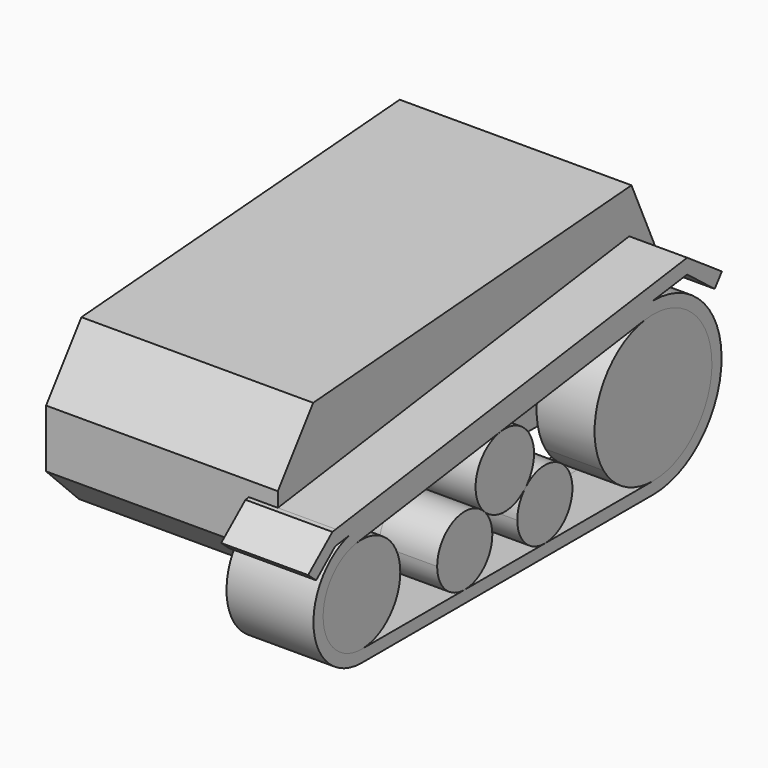
from build123d import *

# Parameters (mm, degrees)
F1_DEPTH      = 40
F3_DEPTH      = 10
F3_DEPTH_BACK = 5
F5_DEPTH      = 5
F6_DEPTH      = 10


# Not quite as in the source:
# - a feature of the source that left no trace in its solid (it failed there, or was rolled back) is left out


with BuildPart() as f1:
    # F0 (on Right) → F1 (new body)
    with BuildSketch(Plane.YZ):
        Polygon((27.6961897601, -10), (38.5682727188, 0), (28.4053542368, 22.532921263), (-40.2577161056, 17.3983419039), (-47.8760995143, 7.0710678119), (-47.8760995143, -2.9289321881), (-40.8050317025, -10), align=None)
    extrude(amount=F1_DEPTH)

    # F4 (on face) → F5 (cut)
    with BuildSketch(Plane.YZ.offset(40)):
        Polygon((33.5502247129, 11.1258671229), (33.3687316656, 11.2501096426), (-47.8760995143, 0), (-47.8760995143, -2.9289321881), (-40.8050317025, -10), (27.6961897601, -10), (38.5682727188, 0), align=None)
    extrude(amount=-F5_DEPTH, mode=Mode.SUBTRACT)


with BuildPart() as f3:
    # F2 (on face) → F3 (new body, two sides)
    with BuildSketch(Plane.YZ.offset(40)) as f3_sk:
        with BuildLine():
            Line((-42.2927111518, 2.7837480747), (20.5938176628, 11.4508923365))
            Line((20.5938176628, 11.4508923365), (27.9149531109, 12.4337729067))
            Line((27.9149531109, 12.4337729067), (33.8481068611, 7.8312940896))
            Line((33.8481068611, 7.8312940896), (34.5993614092, 8.799752374))
            Line((34.5993614092, 8.799752374), (33.5502247129, 11.1258671229))
            Line((33.5502247129, 11.1258671229), (27.9149531109, 14.9835374473))
            Line((27.9149531109, 14.9835374473), (-47.8760995143, 4.5378665025))
            Line((-47.8760995143, 4.5378665025), (-47.8760995143, 2.0142345824))
            Line((-47.8760995143, 2.0142345824), (-45.1088561501, 2.3956214692))
            ThreePointArc((-45.1088561501, 2.3956214692), (-43.7140938337, 2.6862599718), (-42.2927111518, 2.7837480747))
        make_face()
        with BuildLine():
            ThreePointArc((18.8581583186, 9.2408059274), (28.9052740662, 6.2480712147), (33.2478147965, -3.2935919481))
            ThreePointArc((33.2478147965, -3.2935919481), (33.2188858392, -4.1487509974), (33.1322312395, -5))
            Line((33.1322312395, -5), (35.3348394178, -2.9740697466))
            ThreePointArc((35.3348394178, -2.9740697466), (30.9061555825, 7.2446955527), (20.5938176628, 11.4508923365))
            Line((20.5938176628, 11.4508923365), (-42.2927111518, 2.7837480747))
            Line((-42.2927111518, 2.7837480747), (-45.1088561501, 2.3956214692))
            ThreePointArc((-45.1088561501, 2.3956214692), (-46.5376854534, 1.8789836315), (-47.8760995143, 1.159876105))
            Line((-47.8760995143, 1.159876105), (-47.8760995143, -1.4576985119))
            ThreePointArc((-47.8760995143, -1.4576985119), (-45.8111546371, -0.0867559808), (-43.4339984475, 0.6151052728))
            Line((-43.4339984475, 0.6151052728), (-12.2879200079, 4.9279556079))
            Line((-12.2879200079, 4.9279556079), (18.8581583186, 9.2408059274))
        make_face()
        with BuildLine():
            Line((35.3348394178, -2.9740697466), (33.1322312395, -5))
            ThreePointArc((33.1322312395, -5), (28.9164002206, -12.8255520314), (20.5938176628, -15.9475890818))
            Line((20.5938176628, -15.9475890818), (-2.7829632369, -15.9475890818))
            Line((-2.7829632369, -15.9475890818), (-20.0637951493, -15.9475890818))
            Line((-20.0637951493, -15.9475890818), (-42.2927111518, -15.9475890818))
            ThreePointArc((-42.2927111518, -15.9475890818), (-50.056910311, -10.6186987382), (-47.8760995143, -1.4576985119))
            Line((-47.8760995143, -1.4576985119), (-47.8760995143, 1.159876105))
            ThreePointArc((-47.8760995143, 1.159876105), (-52.2891717155, -10.5342898377), (-42.2927111518, -18.0375890818))
            Line((-42.2927111518, -18.0375890818), (20.5938176628, -18.0380762327))
            ThreePointArc((20.5938176628, -18.0380762327), (31.1321051636, -13.6059298678), (35.3348394178, -2.9740697466))
        make_face()
        Polygon((-48.027382516, 1.9933844635), (-47.8760995143, 2.0142345824), (-47.8760995143, 4.5378665025), (-48.6158784645, 4.4359087223), (-53.8486540318, 0), (-52.1195121109, -1.4973431826), align=None)
        Polygon((33.5502247129, 11.1258671229), (34.5993614092, 8.799752374), (35.414042781, 9.8499755317), align=None)
        with BuildLine():
            Line((-45.1088561501, 2.3956214692), (-42.2927111518, 2.7837480747))
            ThreePointArc((-42.2927111518, 2.7837480747), (-43.7140938337, 2.6862599718), (-45.1088561501, 2.3956214692))
        make_face()
    extrude(amount=F3_DEPTH)
    extrude(f3_sk.sketch, amount=-F3_DEPTH_BACK)


with BuildPart() as f3b:
    # F2 (on face) → F3, piece 2 (new body, two sides)
    with BuildSketch(Plane.YZ.offset(40)) as f3_2_sk:
        with BuildLine():
            ThreePointArc((-5.1203578701, -1.3154927046), (-7.2833998095, 3.4372589676), (-12.2879200079, 4.9279556079))
            ThreePointArc((-12.2879200079, 4.9279556079), (-17.401198533, 0.6829450567), (-15.8689310869, -5.7837301576))
            ThreePointArc((-15.8689310869, -5.7837301576), (-11.4233791809, -7.6185140173), (-6.9778272761, -5.783730155))
            ThreePointArc((-6.9778272761, -5.783730155), (-5.603220848, -3.7349626107), (-5.1203578701, -1.3154927046))
        make_face()
    extrude(amount=F3_DEPTH)
    extrude(f3_2_sk.sketch, amount=-F3_DEPTH_BACK)


with BuildPart() as f3c:
    # F2 (on face) → F3, piece 3 (new body, two sides)
    with BuildSketch(Plane.YZ.offset(40)) as f3_3_sk:
        with BuildLine():
            ThreePointArc((-2.7829632369, -15.9475890818), (1.4226173479, -14.2055805787), (3.1646258655, -10))
            Line((3.1646258655, -10), (-8.7305522981, -10))
            ThreePointArc((-8.7305522981, -10), (-6.988543795, -14.2055805642), (-2.7829632369, -15.9475890818))
        make_face()
        with BuildLine():
            Line((-8.7305522981, -10), (3.1646258655, -10))
            ThreePointArc((3.1646258655, -10), (-0.4999292476, -4.5080448123), (-6.9778272761, -5.783730155))
            ThreePointArc((-6.9778272761, -5.783730155), (-8.274918404, -7.7169660313), (-8.7305522981, -10))
        make_face()
    extrude(amount=F3_DEPTH)
    extrude(f3_3_sk.sketch, amount=-F3_DEPTH_BACK)


with BuildPart() as f3d:
    # F2 (on face) → F3, piece 4 (new body, two sides)
    with BuildSketch(Plane.YZ.offset(40)) as f3_4_sk:
        with BuildLine():
            ThreePointArc((-20.0637951493, -15.9475890818), (-15.8582145779, -14.2055805715), (-14.1162060675, -10))
            Line((-14.1162060675, -10), (-26.0113842311, -10))
            ThreePointArc((-26.0113842311, -10), (-24.2693757208, -14.2055805715), (-20.0637951493, -15.9475890818))
        make_face()
        with BuildLine():
            ThreePointArc((-14.1162060675, -10), (-14.5718399609, -7.7169660331), (-15.8689310869, -5.7837301576))
            ThreePointArc((-15.8689310869, -5.7837301576), (-22.3468291163, -4.5080448116), (-26.0113842311, -10))
            Line((-26.0113842311, -10), (-14.1162060675, -10))
        make_face()
    extrude(amount=F3_DEPTH)
    extrude(f3_4_sk.sketch, amount=-F3_DEPTH_BACK)


with BuildPart() as f6:
    # F2 (on face) → F6 (new body)
    with BuildSketch(Plane.YZ.offset(40)):
        with BuildLine():
            ThreePointArc((-33.9720425736, -7.6269205036), (-36.8274914742, -1.3527751861), (-43.4339984475, 0.6151052728))
            ThreePointArc((-43.4339984475, 0.6151052728), (-45.8111546371, -0.0867559808), (-47.8760995143, -1.4576985119))
            Line((-47.8760995143, -1.4576985119), (-47.8760995143, -2.9289321881))
            Line((-47.8760995143, -2.9289321881), (-40.8050317025, -10))
            Line((-40.8050317025, -10), (-34.3176237359, -10))
            ThreePointArc((-34.3176237359, -10), (-34.0588911131, -8.8259756145), (-33.9720425736, -7.6269205036))
        make_face()
        with BuildLine():
            Line((-47.8760995143, -2.9289321881), (-47.8760995143, -1.4576985119))
            ThreePointArc((-47.8760995143, -1.4576985119), (-50.056910311, -10.6186987382), (-42.2927111518, -15.9475890818))
            ThreePointArc((-42.2927111518, -15.9475890818), (-37.3183811673, -14.296970488), (-34.3176237359, -10))
            Line((-34.3176237359, -10), (-40.8050317025, -10))
            Line((-40.8050317025, -10), (-47.8760995143, -2.9289321881))
        make_face()
    extrude(amount=F6_DEPTH)


with BuildPart() as f6b:
    # F2 (on face) → F6, piece 2 (new body)
    with BuildSketch(Plane.YZ.offset(40)):
        with BuildLine():
            ThreePointArc((20.5938176628, -15.9475890818), (28.9164002206, -12.8255520314), (33.1322312395, -5))
            Line((33.1322312395, -5), (27.6961897601, -10))
            Line((27.6961897601, -10), (9.8631264222, -10))
            ThreePointArc((9.8631264222, -10), (14.4594564412, -14.3612590854), (20.5938176628, -15.9475890818))
        make_face()
        with BuildLine():
            ThreePointArc((33.1322312395, -5), (33.2188858392, -4.1487509974), (33.2478147965, -3.2935919481))
            ThreePointArc((33.2478147965, -3.2935919481), (28.9052740662, 6.2480712147), (18.8581583186, 9.2408059274))
            ThreePointArc((18.8581583186, 9.2408059274), (9.1306319184, 2.0654206522), (9.8631264222, -10))
            Line((9.8631264222, -10), (27.6961897601, -10))
            Line((27.6961897601, -10), (33.1322312395, -5))
        make_face()
    extrude(amount=F6_DEPTH)


solid = Compound([f1.part, f3.part, f3b.part, f3c.part, f3d.part, f6.part, f6b.part])
